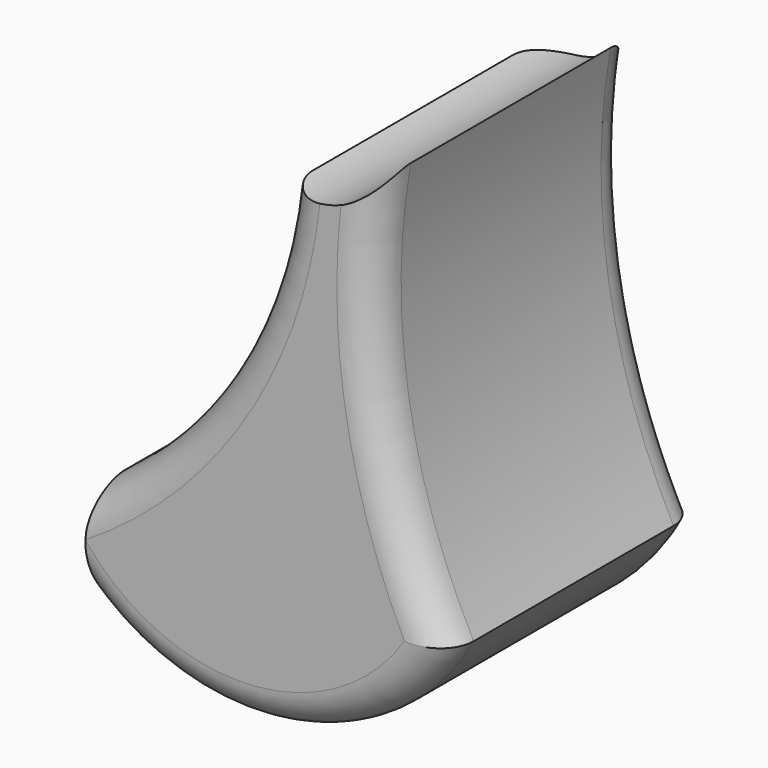
from build123d import *

# Parameters (mm, degrees)
F1_DEPTH    = 9
F2_T2_ANGLE = 69.5952889026
F2_T4_ANGLE = 54.4883301746
F2_T6_ANGLE = 143.7551987737
F3_R        = 1


# Not quite as in the source:
# - a fillet or chamfer that OpenCascade refuses, or shapes differently, is made with other operations: its cross-section is extruded or revolved along the edge and cut away or added


with BuildPart() as f1:
    # F0 (on Front) → F1 (new body)
    with BuildSketch(Plane.XZ):
        with BuildLine():
            ThreePointArc((14.7663247772, 11.9293080643), (12.944509625, 17.3914763041), (13.0025018007, 23.1491606683))
            ThreePointArc((13.0025018007, 23.1491606683), (11.8204746449, 22.132281974), (10.26218878, 22.0777325565))
            ThreePointArc((10.26218878, 22.0777325565), (8.5829178564, 16.9649844736), (4.9823031081, 12.9655198559))
            ThreePointArc((4.9823031081, 12.9655198559), (4.6861100149, 11.4138618351), (4.9823031081, 9.8622038143))
            ThreePointArc((4.9823031081, 9.8622038143), (10.3556125988, 8.6176722475), (14.7663247772, 11.9293080643))
        make_face()
    extrude(amount=F1_DEPTH)

    # F2: fillet of radius 1 on 3 edges, made by hand

    # F2_s1 → F2_t2 (revolve, cut)
    with BuildSketch(Plane(origin=(-1.9409501927, 0, 23.5660641142), x_dir=(0, 1, 0), z_dir=(-0.0820841468, 0, 0.9966254025))):
        with BuildLine():
            ThreePointArc((-8, -12.2787262208), (-8.7071067812, -12.5716194396), (-9, -13.2787262208))
            Line((-9, -13.2787262208), (-9, -12.2787262208))
            Line((-9, -12.2787262208), (-8, -12.2787262208))
        make_face()
    revolve(axis=Axis((-2.70136938, -9, 23.5034344039), (0, 1, 0)), revolution_arc=F2_T2_ANGLE, mode=Mode.SUBTRACT)

    # F2_s3 → F2_t4 (revolve, cut)
    with BuildSketch(Plane(origin=(0.9320888174, 0, -1.2745523028), x_dir=(0, 1, 0), z_dir=(0.5902994367, 0, -0.8071843501))):
        with BuildLine():
            ThreePointArc((-8, 18.7819322745), (-8.7071067812, 18.4890390557), (-9, 17.7819322745))
            Line((-9, 17.7819322745), (-9, 18.7819322745))
            Line((-9, 18.7819322745), (-8, 18.7819322745))
        make_face()
    revolve(axis=Axis((30.156216129, -9, 20.0972519028), (0, 1, 0)), revolution_arc=F2_T4_ANGLE, mode=Mode.SUBTRACT)

    # F2_s5 → F2_t6 (revolve, cut)
    with BuildSketch(Plane(origin=(-4.2476398352, 0, 7.3417188573), x_dir=(0, 1, 0), z_dir=(-0.5007864485, 0, 0.8655708712))):
        with BuildLine():
            ThreePointArc((-8, -8.7783825872), (-8.7071067812, -9.071275806), (-9, -9.7783825872))
            Line((-9, -9.7783825872), (-9, -8.7783825872))
            Line((-9, -8.7783825872), (-8, -8.7783825872))
        make_face()
    revolve(axis=Axis((9.0052261238, -9, 15.0093240152), (0, -1, 0)), revolution_arc=F2_T6_ANGLE, mode=Mode.SUBTRACT)

    # F3#2 (call 1 of 2: OpenCascade refuses the feature's edges together)
    f3_2_edges = [f1.edges().sort_by_distance(p)[0] for p in [
        (8.582918, 0, 16.964984),
    ]]
    fillet(f3_2_edges, radius=F3_R)

    # F3 (call 2 of 2)
    f3_edges = [f1.edges().sort_by_distance(p)[0] for p in [
        (12.94451, 0, 17.391476),
        (10.355613, 0, 8.617672),
    ]]
    fillet(f3_edges, radius=F3_R)


solid = f1.part
